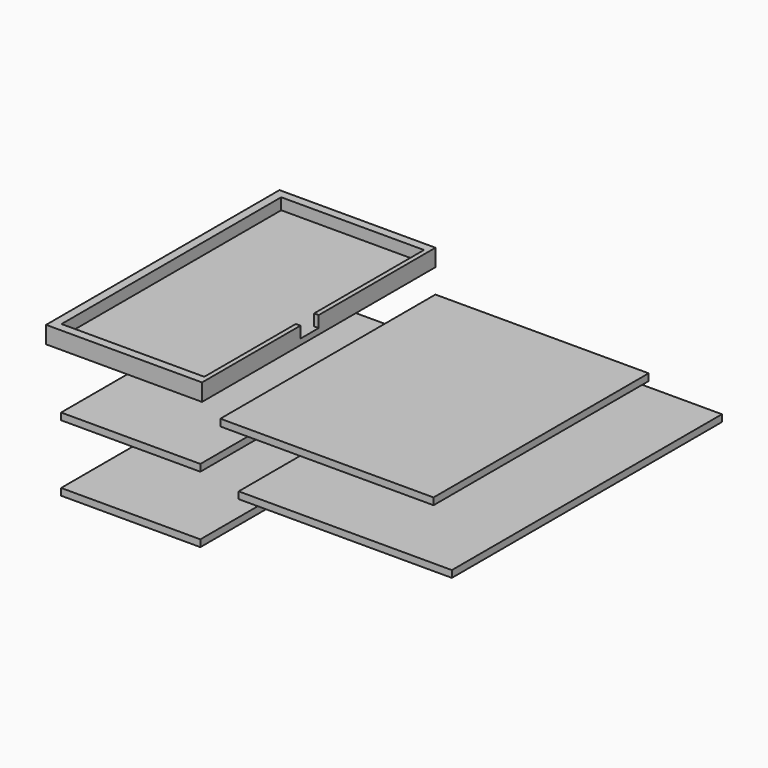
from build123d import *

# Parameters (mm, degrees)
F1_DEPTH  = 500
F2_W      = 6810
F2_H      = 12740
F3_DEPTH  = 250
F6_W      = 6080
F6_H      = 12010
F7_DEPTH  = 300
F9_W      = 6080
F9_H      = 12010
F10_DEPTH = 300
F13_DEPTH = 300
F15_W     = 9310
F15_H     = 11740
F16_DEPTH = 300


# Not quite as in the source:
# - a feature names something its author has since deleted; it is built from what else it names


with BuildPart() as f1:
    # F0 (on Top) → F1 (new body)
    with BuildSketch(Plane.XY):
        Polygon((0, 0), (0, 6370), (-6810, 6370), (-6810, -6370), (0, -6370), (0, -1000), (-200, -1000), (-200, -5995), (-6435, -5995), (-6435, 5995), (-200, 5995), (-200, 0), align=None)
    extrude(amount=F1_DEPTH)

    # F2 (on Top) → F3 (join)
    with BuildSketch(Plane.XY):
        with Locations((-3405, 0)):
            Rectangle(F2_W, F2_H)
    extrude(amount=-F3_DEPTH)


with BuildPart() as f7:
    # F6 (on offset) → F7 (new body)
    with BuildSketch(Plane.XY.offset(-2900)):
        with Locations((-3405, 0)):
            Rectangle(F6_W, F6_H)
    extrude(amount=-F7_DEPTH)


with BuildPart() as f10:
    # F9 (on offset) → F10 (new body)
    with BuildSketch(Plane(origin=(0, 0, -5800), x_dir=(1, 0, 0), z_dir=(0, 0, -1))):
        with Locations((-3405, 0)):
            Rectangle(F9_W, F9_H)
    extrude(amount=F10_DEPTH)


with BuildPart() as f13:
    # F12 (on offset) → F13 (new body)
    with BuildSketch(Plane.XY.offset(-4500)):
        Polygon((4000, 4870), (0, 4870), (0, -4370), (9310, -4370), (9310, 10370), (4000, 10370), align=None)
    extrude(amount=-F13_DEPTH)


with BuildPart() as f16:
    # F15 (on offset) → F16 (new body)
    with BuildSketch(Plane.XY.offset(-1300)):
        with Locations((4655, 500)):
            Rectangle(F15_W, F15_H)
    extrude(amount=-F16_DEPTH)


solid = Compound([f1.part, f7.part, f10.part, f13.part, f16.part])
